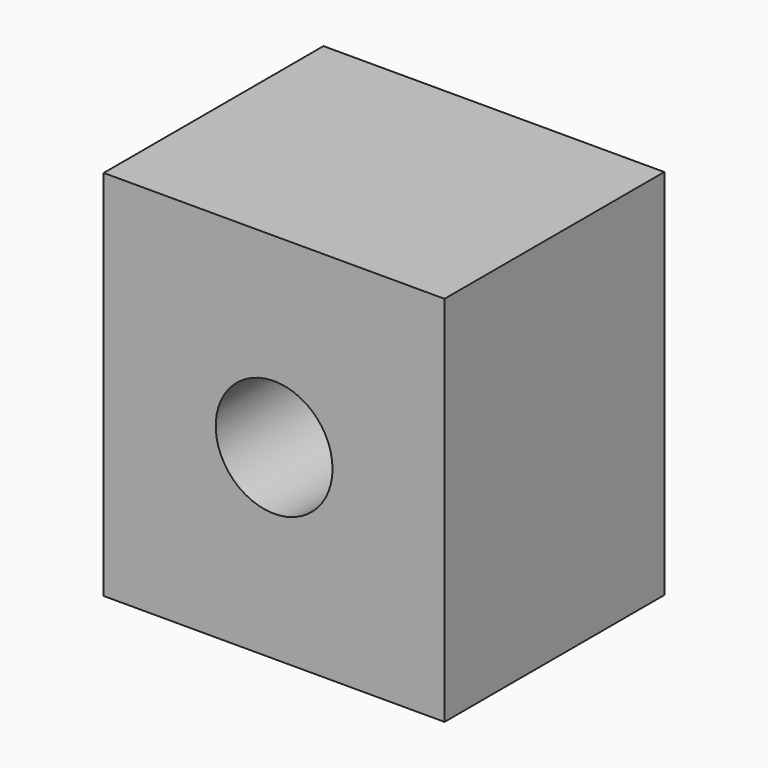
from build123d import *

# Parameters (mm, degrees)
F0_W     = 31.5161347389
F0_H     = 34.4433300197
F0_R     = 5.3996855878
F1_DEPTH = 25.4


# Not quite as in the source:
# - the program builds the solid bodies; features that only make, move or delete a surface that nothing else refers to are left out


with BuildPart() as f1:
    # F0 (on Front) → F1 (new body)
    with BuildSketch(Plane.XZ):
        Rectangle(F0_W, F0_H)
        Circle(F0_R, mode=Mode.SUBTRACT)
    extrude(amount=F1_DEPTH)


solid = f1.part
